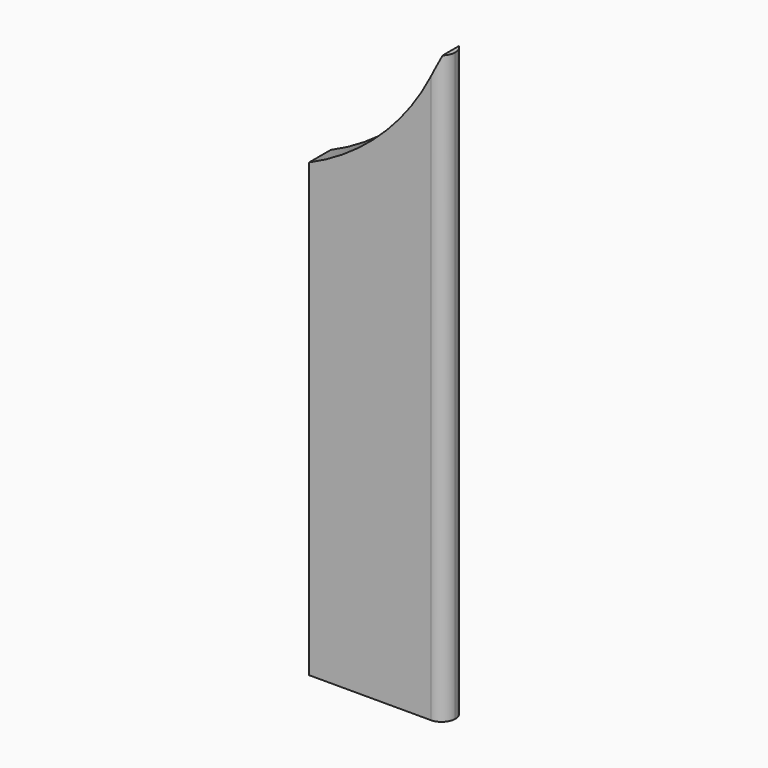
from build123d import *

# Parameters (mm, degrees)
F1_DEPTH = 12
F2_R     = 5.99999


# Not quite as in the source:
# - a fillet or chamfer is up to 0.001 mm smaller than in the source, because OpenCascade refuses the exact size


with BuildPart() as f1:
    # F0 (on Front) → F1 (new body)
    with BuildSketch(Plane.XZ):
        with BuildLine():
            Line((0, 200), (0, 0))
            Line((0, 0), (60, 0))
            Line((60, 0), (60, 260))
            Line((60, 260), (58, 260))
            ThreePointArc((58, 260), (34.9106792543, 224.2863433875), (0, 200))
        make_face()
    extrude(amount=F1_DEPTH)

    # F2 (radius 6 in the source; OpenCascade refuses exactly that, so slightly less here)
    f2_edges = [f1.edges().sort_by_distance(p)[0] for p in [
        (60, -12, 130),
        (60, 0, 130),
    ]]
    fillet(f2_edges, radius=F2_R)


solid = f1.part
